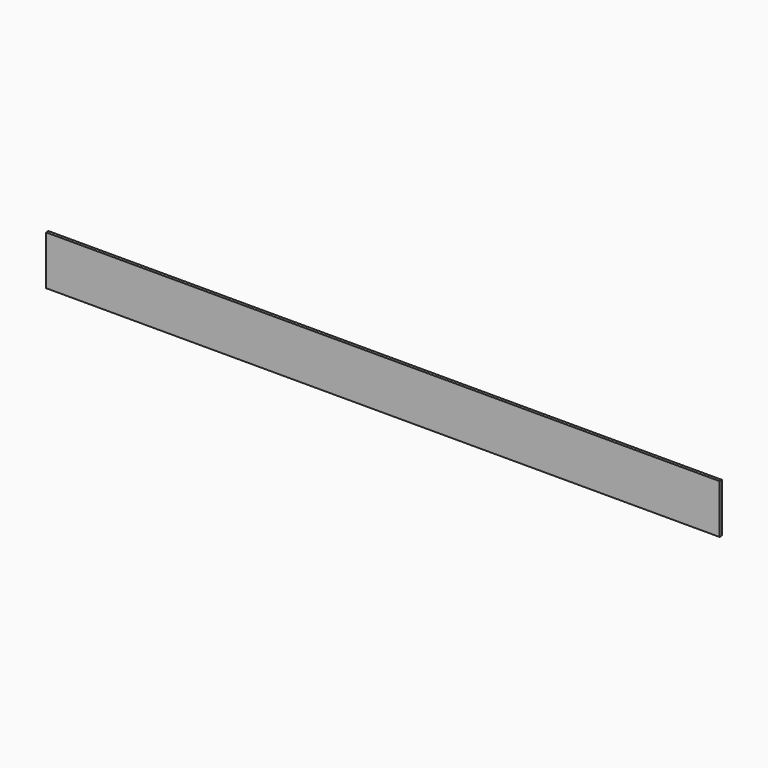
from build123d import *

# Parameters (mm, degrees)
F0_W     = 584.2
F0_H     = 42.6317787108
F1_DEPTH = 2.54


# Not quite as in the source:
# - a length typed as a fraction of an inch, garbled in the dataset ("3 / 203.2 mm" for 3/8 in), is restored


with BuildPart() as f1:
    # F0 (on Front) → F1 (new body)
    with BuildSketch(Plane.XZ):
        with Locations((292.1, 21.3158893554)):
            Rectangle(F0_W, F0_H)
    extrude(amount=F1_DEPTH)


solid = f1.part
